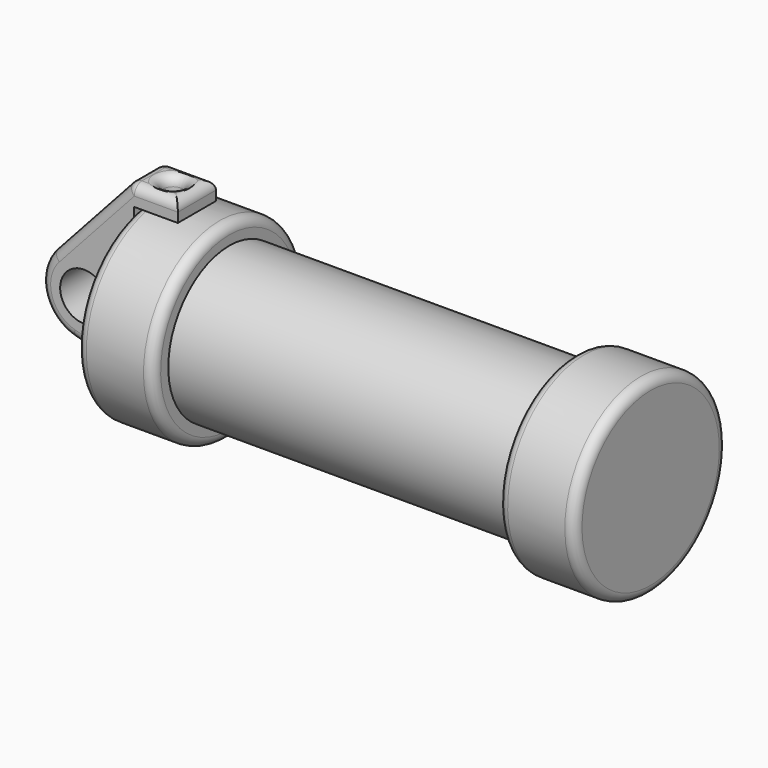
from build123d import *

# Parameters (mm, degrees)
F0_W           = 5.842
F0_H           = 12.7
F0_R           = 3.175
F2_DEPTH       = 3.175
F5_D           = 2.54
F5_2_D         = 2.54
F6_F1_R        = 1.27
F6_F2_R        = 1.27
F6_F3_R        = 1.27
F6_F4_R        = 1.27
F6_2_T1_DEPTH  = 8.9637681337
F6_2_T3_DEPTH  = 14.8458939279
F6_2_T5_DEPTH  = 17.7294216388
F6_2_T7_DEPTH  = 12.7
F6_2_T9_DEPTH  = 3.81
F6_2_T14_DEPTH = 1.27
F6_2_T20_DEPTH = 1.27
F6_2_T24_ANGLE = 116.8111069241
F6_2_T26_ANGLE = 116.8111069241


# Not quite as in the source:
# - a fillet or chamfer that OpenCascade refuses, or shapes differently, is made with other operations: its cross-section is extruded or revolved along the edge and cut away or added


with BuildPart() as f1:
    # F0 (on Front) → F1 (revolve)
    with BuildSketch(Plane.XZ):
        Polygon((5.842, 12.7), (5.842, 0), (66.294, 0), (66.294, 12.7), (56.134, 12.7), (56.134, 10.16), (10.16, 10.16), (10.16, 12.7), align=None)
        with Locations((2.921, 6.35)):
            Rectangle(F0_W, F0_H)
    revolve(axis=Axis((33.147, 0, 0), (-1, 0, 0)))

    # F5 (through all)
    with Locations(Plane.XY.offset(15.24)):
        with Locations((2.667, 0)):
            Hole(F5_D / 2)

    # F6: fillet of radius 1.27 on 4 edges, made by hand

    # F6_f1
    f6_f1_edges = [f1.edges().sort_by_distance(p)[0] for p in [
        (66.294, 0, -12.7),
    ]]
    fillet(f6_f1_edges, radius=F6_F1_R)

    # F6_f2
    f6_f2_edges = [f1.edges().sort_by_distance(p)[0] for p in [
        (56.134, 0, -12.7),
    ]]
    fillet(f6_f2_edges, radius=F6_F2_R)

    # F6_f3
    f6_f3_edges = [f1.edges().sort_by_distance(p)[0] for p in [
        (10.16, 0, -12.7),
    ]]
    fillet(f6_f3_edges, radius=F6_F3_R)

    # F6_f4
    f6_f4_edges = [f1.edges().sort_by_distance(p)[0] for p in [
        (0, 0, -12.7),
    ]]
    fillet(f6_f4_edges, radius=F6_F4_R)


with BuildPart() as f2:
    # F0 (on Front) → F2 (new body, symmetric)
    with BuildSketch(Plane.XZ):
        with BuildLine():
            Line((-0.9398, 0), (0, 0))
            Line((0, 0), (0, 12.7))
            Line((0, 12.7), (5.842, 12.7))
            Line((5.842, 12.7), (5.842, 15.24))
            Line((5.842, 15.24), (-0.508, 15.24))
            Line((-0.508, 15.24), (-10.8806298187, 3.8475430269))
            ThreePointArc((-10.8806298187, 3.8475430269), (-4.5919612295, 5.3297205562), (-0.9398, 0))
        make_face()
        with BuildLine():
            ThreePointArc((-8.1826630726, -5.5069827884), (-3.1957909266, -4.5493385486), (-0.9398, 0))
            ThreePointArc((-0.9398, 0), (-4.5919612295, 5.3297205562), (-10.8806298187, 3.8475430269))
            ThreePointArc((-10.8806298187, 3.8475430269), (-12.1459778134, -1.5837270034), (-8.1826630726, -5.5069827884))
        make_face()
        with Locations((-6.6548, 0)):
            Circle(F0_R, mode=Mode.SUBTRACT)
        with BuildLine():
            Line((5.842, 0), (0, 0))
            Line((0, 0), (-0.9398, 0))
            ThreePointArc((-0.9398, 0), (-3.1957909266, -4.5493385486), (-8.1826630726, -5.5069827884))
            Line((-8.1826630726, -5.5069827884), (5.842, -9.398))
            Line((5.842, -9.398), (5.842, 0))
        make_face()
    extrude(amount=F2_DEPTH, both=True)

    # F5#2 (through all)
    with Locations(Plane.XY.offset(15.24)):
        with Locations((2.667, 0)):
            Hole(F5_2_D / 2)

    # F6#2: fillet of radius 1.27 on 11 edges, made by hand

    # F6_2_s2 → F6_2_t1 (cut)
    with BuildSketch(Plane.YZ.offset(0.0532318663)):
        with BuildLine():
            ThreePointArc((-3.175, 13.97), (-2.8030256121, 14.8680256121), (-1.905, 15.24))
            Line((-1.905, 15.24), (-3.175, 15.24))
            Line((-3.175, 15.24), (-3.175, 13.97))
        make_face()
        with BuildLine():
            ThreePointArc((3.175, 13.97), (2.8030256121, 14.8680256121), (1.905, 15.24))
            Line((1.905, 15.24), (3.175, 15.24))
            Line((3.175, 15.24), (3.175, 13.97))
        make_face()
    extrude(amount=F6_2_T1_DEPTH, mode=Mode.SUBTRACT)

    # F6_2_s4 → F6_2_t3 (cut)
    with BuildSketch(Plane(origin=(6.9785232931, 0, 7.6646451037), x_dir=(0, 1, 0), z_dir=(-0.6732358752, 0, -0.7394277898))):
        with BuildLine():
            ThreePointArc((-3.175, -9.3657440555), (-2.8030256121, -10.2637696676), (-1.905, -10.6357440555))
            Line((-1.905, -10.6357440555), (-3.175, -10.6357440555))
            Line((-3.175, -10.6357440555), (-3.175, -9.3657440555))
        make_face()
        with BuildLine():
            ThreePointArc((3.175, -9.3657440555), (2.8030256121, -10.2637696676), (1.905, -10.6357440555))
            Line((1.905, -10.6357440555), (3.175, -10.6357440555))
            Line((3.175, -10.6357440555), (3.175, -9.3657440555))
        make_face()
    extrude(amount=F6_2_T3_DEPTH, mode=Mode.SUBTRACT)

    # F6_2_s6 → F6_2_t5 (cut)
    with BuildSketch(Plane(origin=(-6.179167626, 0, 1.7143547379), x_dir=(0, 1, 0), z_dir=(0.9636015378, 0, -0.2673426199))):
        with BuildLine():
            ThreePointArc((-3.175, -6.2241116667), (-2.8030256121, -7.1221372788), (-1.905, -7.4941116667))
            Line((-1.905, -7.4941116667), (-3.175, -7.4941116667))
            Line((-3.175, -7.4941116667), (-3.175, -6.2241116667))
        make_face()
        with BuildLine():
            ThreePointArc((3.175, -6.2241116667), (2.8030256121, -7.1221372788), (1.905, -7.4941116667))
            Line((1.905, -7.4941116667), (3.175, -7.4941116667))
            Line((3.175, -7.4941116667), (3.175, -6.2241116667))
        make_face()
    extrude(amount=F6_2_T5_DEPTH, mode=Mode.SUBTRACT)

    # F6_2_s8 → F6_2_t7 (cut)
    with BuildSketch(Plane.XZ.offset(-6.35)):
        with BuildLine():
            ThreePointArc((5.842, 13.97), (5.4700256121, 14.8680256121), (4.572, 15.24))
            Line((4.572, 15.24), (5.842, 15.24))
            Line((5.842, 15.24), (5.842, 13.97))
        make_face()
    extrude(amount=F6_2_T7_DEPTH, mode=Mode.SUBTRACT)

    # F6_2_s10 → F6_2_t9 (cut)
    with BuildSketch(Plane.XZ.offset(-1.905)):
        with BuildLine():
            ThreePointArc((0.0532318663, 15.24), (-0.4601090812, 15.1316286289), (-0.8858414267, 14.8250095615))
            Line((-0.8858414267, 14.8250095615), (-0.508, 15.24))
            Line((-0.508, 15.24), (0.0532318663, 15.24))
        make_face()
    extrude(amount=F6_2_T9_DEPTH, mode=Mode.SUBTRACT)


with BuildPart() as f6_2_tool12:
    # F6_2_s13 → F6_2_t14 (new body)
    with BuildSketch(Plane.XZ.offset(1.905)):
        Polygon((0.0532318663, 13.97), (0.0532318663, 15.24), (-0.508, 15.24), (-0.8858414267, 14.8250095615), align=None)
    extrude(amount=F6_2_T14_DEPTH)

    # F6_2_s15 → F6_2_t16 (revolve, cut)
    with BuildSketch(Plane(origin=(0.0532318663, -1.905, 13.97), x_dir=(0.4042054705, 0, -0.9146682118), z_dir=(-0.9146682118, 0, -0.4042054705))):
        with BuildLine():
            ThreePointArc((0, -1.27), (1.27, 0), (0, 1.27))
            Line((0, 1.27), (0, -1.27))
        make_face()
    revolve(axis=Axis((0.0532318663, -1.905, 13.97), (0, -1, 0)), mode=Mode.SUBTRACT)


with BuildPart() as f2_1:
    add(f2.part)

    # F6_2_t11: cut F6_2_tool12
    add(f6_2_tool12.part, mode=Mode.SUBTRACT)


with BuildPart() as f6_2_tool18:
    # F6_2_s19 → F6_2_t20 (new body)
    with BuildSketch(Plane.XZ.offset(-1.905)):
        Polygon((0.0532318663, 13.97), (0.0532318663, 15.24), (-0.508, 15.24), (-0.8858414267, 14.8250095615), align=None)
    extrude(amount=-F6_2_T20_DEPTH)

    # F6_2_s21 → F6_2_t22 (revolve, cut)
    with BuildSketch(Plane(origin=(0.0532318663, 1.905, 13.97), x_dir=(0.4042054705, 0, -0.9146682118), z_dir=(0.9146682118, 0, 0.4042054705))):
        with BuildLine():
            ThreePointArc((0, -1.27), (1.27, 0), (0, 1.27))
            Line((0, 1.27), (0, -1.27))
        make_face()
    revolve(axis=Axis((0.0532318663, 1.905, 13.97), (0, 1, 0)), mode=Mode.SUBTRACT)


with BuildPart() as f2_2:
    add(f2_1.part)

    # F6_2_t17: cut F6_2_tool18
    add(f6_2_tool18.part, mode=Mode.SUBTRACT)

    # F6_2_s23 → F6_2_t24 (revolve, cut)
    with BuildSketch(Plane(origin=(-3.0162650989, 0, -3.3128214309), x_dir=(0, 1, 0), z_dir=(0.6732358752, 0, 0.7394277898))):
        with BuildLine():
            ThreePointArc((-3.175, 9.3657440555), (-2.8030256121, 10.2637696676), (-1.905, 10.6357440555))
            Line((-1.905, 10.6357440555), (-3.175, 10.6357440555))
            Line((-3.175, 10.6357440555), (-3.175, 9.3657440555))
        make_face()
    revolve(axis=Axis((-6.6548, -3.175, 0), (0, -1, 0)), revolution_arc=F6_2_T24_ANGLE, mode=Mode.SUBTRACT)

    # F6_2_s25 → F6_2_t26 (revolve, cut)
    with BuildSketch(Plane(origin=(-3.0162650989, 0, -3.3128214309), x_dir=(0, 1, 0), z_dir=(0.6732358752, 0, 0.7394277898))):
        with BuildLine():
            ThreePointArc((3.175, 9.3657440555), (2.8030256121, 10.2637696676), (1.905, 10.6357440555))
            Line((1.905, 10.6357440555), (3.175, 10.6357440555))
            Line((3.175, 10.6357440555), (3.175, 9.3657440555))
        make_face()
    revolve(axis=Axis((-6.6548, 3.175, 0), (0, -1, 0)), revolution_arc=F6_2_T26_ANGLE, mode=Mode.SUBTRACT)

    # F6_2_s27 → F6_2_t28 (revolve, cut)
    with BuildSketch(Plane.XZ):
        with BuildLine():
            ThreePointArc((5.207, 15.24), (4.3089743879, 14.8680256121), (3.937, 13.97))
            Line((3.937, 13.97), (3.937, 15.24))
            Line((3.937, 15.24), (5.207, 15.24))
        make_face()
    revolve(axis=Axis((2.667, 0, 15.24), (0, 0, 1)), mode=Mode.SUBTRACT)


solid = Compound([f1.part, f2_2.part])
